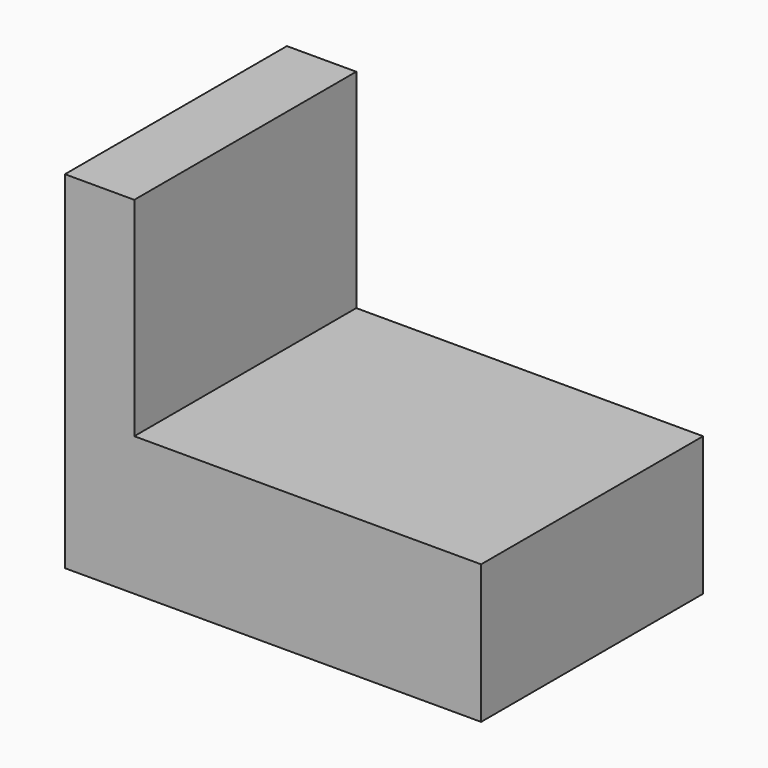
from build123d import *

# Parameters (mm, degrees)
F1_DEPTH = 12.7


# Not quite as in the source:
# - a feature names something its author has since deleted; it is built from what else it names


with BuildPart() as f1:
    # F0 (on Front) → F1 (new body, symmetric)
    with BuildSketch(Plane.XZ):
        Polygon((0, 31.75), (0, 0), (38.1, 0), (38.1, 12.7), (6.35, 12.7), (6.35, 31.75), align=None)
    extrude(amount=F1_DEPTH, both=True)


solid = f1.part
